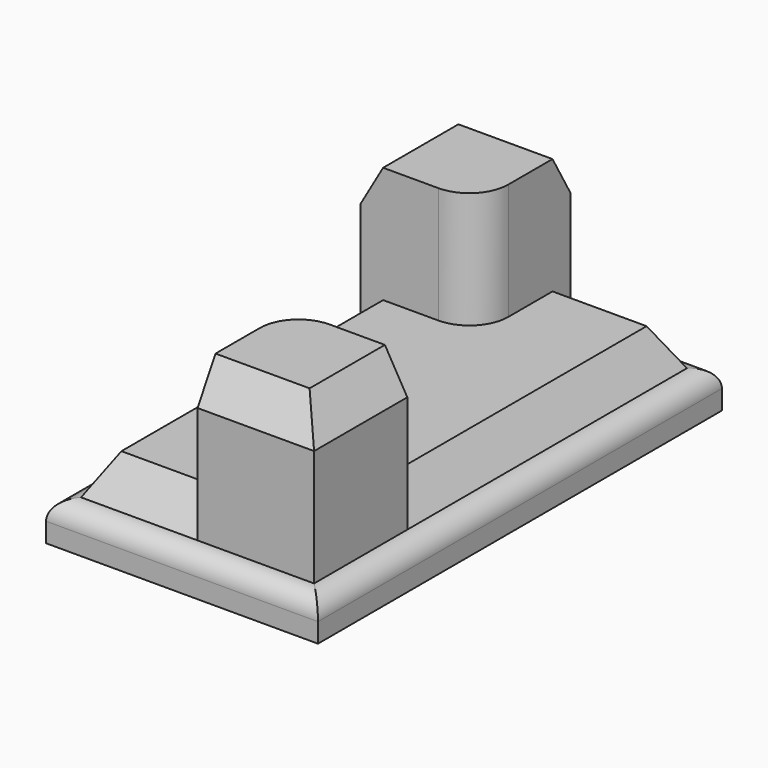
from build123d import *

# Parameters (mm, degrees)
F0_W     = 88.9000000224
F0_H     = 165.1000027703
F1_DEPTH = 12.7
F2_DEPTH = 25.4
F3_DEPTH = 63.5
F4_R     = 6.34999
F5_SIZE2 = 7.332338
F5_SIZE  = 12.69999


# Not quite as in the source:
# - a fillet or chamfer is up to 0.001 mm smaller than in the source, because OpenCascade refuses the exact size


with BuildPart() as f1:
    # F0 (on Top) → F1 (new body)
    with BuildSketch(Plane.XY):
        with Locations((38.1000000112, -1.3851e-06)):
            Rectangle(F0_W, F0_H)
        Polygon((0, 38.1), (0, 76.2), (38.1, 76.2), (76.2, 76.2), (76.2, -38.1), (76.2, -76.2), (38.1, -76.2), (0, -76.2), align=None, mode=Mode.SUBTRACT)
    extrude(amount=F1_DEPTH)

    # F0 (on Top) → F2 (join)
    with BuildSketch(Plane.XY):
        with BuildLine():
            Line((25.4, 38.1), (0, 38.1))
            Line((0, 38.1), (0, -76.2))
            Line((0, -76.2), (38.1, -76.2))
            Line((38.1, -76.2), (38.1, -50.8))
            ThreePointArc((38.1, -50.8), (41.8197438789, -41.8197438789), (50.8, -38.1))
            Line((50.8, -38.1), (76.2, -38.1))
            Line((76.2, -38.1), (76.2, 76.2))
            Line((76.2, 76.2), (38.1, 76.2))
            Line((38.1, 76.2), (38.1, 50.8))
            ThreePointArc((38.1, 50.8), (34.3802561211, 41.8197438789), (25.4, 38.1))
        make_face()
    extrude(amount=F2_DEPTH)

    # F0 (on Top) → F3 (join)
    with BuildSketch(Plane.XY):
        with BuildLine():
            Line((38.1, 76.2), (0, 76.2))
            Line((0, 76.2), (0, 38.1))
            Line((0, 38.1), (25.4, 38.1))
            ThreePointArc((25.4, 38.1), (34.3802561211, 41.8197438789), (38.1, 50.8))
            Line((38.1, 50.8), (38.1, 76.2))
        make_face()
        with BuildLine():
            Line((38.1, -50.8), (38.1, -76.2))
            Line((38.1, -76.2), (76.2, -76.2))
            Line((76.2, -76.2), (76.2, -38.1))
            Line((76.2, -38.1), (50.8, -38.1))
            ThreePointArc((50.8, -38.1), (41.8197438789, -41.8197438789), (38.1, -50.8))
        make_face()
    extrude(amount=F3_DEPTH)

    # F4 (radius 6.35 in the source; OpenCascade refuses exactly that, so slightly less here)
    f4_edges = [f1.edges().sort_by_distance(p)[0] for p in [
        (-6.35, -1e-06, 12.7),
        (38.1, -82.550003, 12.7),
        (82.55, -1e-06, 12.7),
        (38.1, 82.55, 12.7),
    ]]
    fillet(f4_edges, radius=F4_R)

    # F5 (size 12.7 and 7.3323484187 in the source; OpenCascade refuses exactly that, so slightly less here)
    f5_edges = [f1.edges().sort_by_distance(p)[0] for p in [
        (57.15, 76.2, 25.4),
        (76.2, 19.05, 25.4),
        (0, -19.05, 25.4),
        (19.05, -76.2, 25.4),
        (57.15, -76.2, 63.5),
        (76.2, -57.15, 63.5),
        (19.05, 76.2, 63.5),
        (0, 57.15, 63.5),
    ]]
    chamfer(f5_edges, length=F5_SIZE, length2=F5_SIZE2)


solid = f1.part
